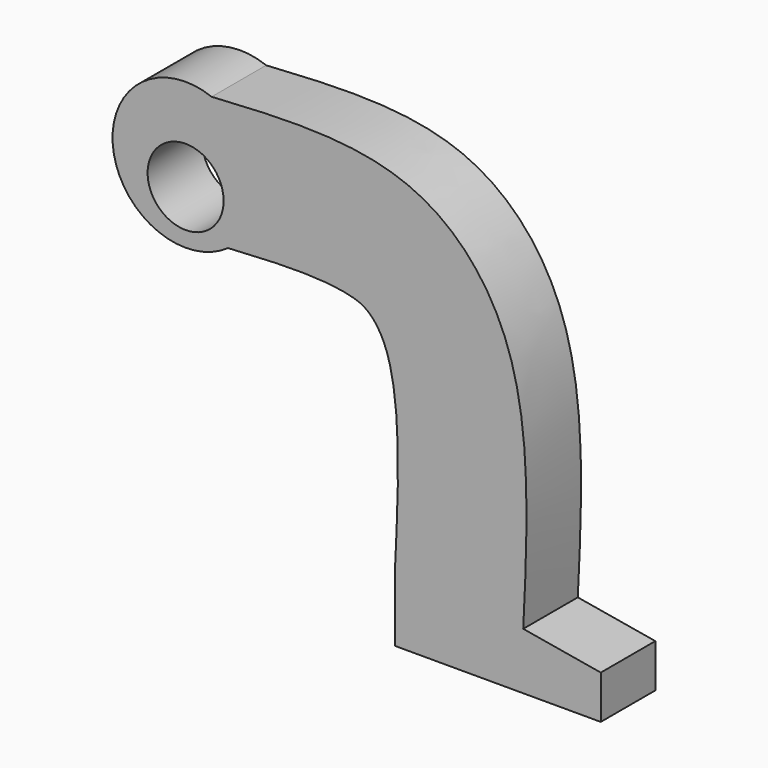
from build123d import *

# Parameters (mm, degrees)
F1_DEPTH = 7
F2_R     = 3.9
F3_DEPTH = 25


# Not quite as in the source:
# - ends of sketch curves that miss each other by under 0.0002 mm in the source are joined
# - the dataset's text gives a spline's control points without its knots; the knots are read off the source's solid


with BuildPart() as f1:
    # F0 (on Front) → F1 (new body)
    with BuildSketch(Plane.XZ):
        with BuildLine():
            add(Edge.make_bspline(
                [(2.6675548526, 7.0095756725), (9.9466486375, 7.453696747), (23.6105158189, 8.2821493946), (35.8507052692, -5.7834758803), (35.0790148845, -21.7545178271), (34.6487350762, -30.6607671082)],
                knots=[0, 0, 0, 0, 0.3351894082, 0.6292627681, 1, 1, 1, 1], degree=3))
            ThreePointArc((2.6675548526, 7.0095756725), (-7.4394221806, -0.9513136277), (4.3455710058, -6.1127745446))
            add(Edge.make_bspline(
                [(4.3455710058, -6.1127745446), (5.3891405614, -6.0498316594), (7.6843362497, -5.9165406912), (10.9253144196, -5.8060227215), (13.8856209942, -5.8700018706), (15.7808027565, -6.0874058733), (16.7453601396, -6.2897087839), (17.1897220211, -6.4084184169), (17.469776248, -6.4959038726), (17.6984548015, -6.5789229449), (17.935730162, -6.6779012945), (18.2137061971, -6.8183248013), (18.5218848655, -7.0140479544), (18.8233111562, -7.2486234624), (19.1262983711, -7.5344088665), (19.4349362667, -7.884892544), (19.7479207593, -8.3124495536), (20.0600135431, -8.8274515425), (20.3124903035, -9.3357541203), (20.505036356, -9.7925679397), (20.6431005208, -10.1598390415), (20.7745963912, -10.5550369644), (20.9490677171, -11.1507905059), (21.1559433245, -12.0126577006), (21.3728446832, -13.2297306672), (21.6070152211, -15.0773377917), (21.7818347688, -17.7706509611), (21.8035125183, -21.4920595704), (21.6778381248, -25.593639044), (21.5366515935, -28.5223388593), (21.4641132996, -30.0237900428)],
                knots=[0.0135442019, 0.0135442019, 0.0135442019, 0.0135442019, 0.0625, 0.125, 0.1875, 0.25, 0.28125, 0.296875, 0.3125, 0.328125, 0.34375, 0.375, 0.40625, 0.4375, 0.46875, 0.5, 0.53125, 0.5625, 0.59375, 0.609375, 0.625, 0.640625, 0.65625, 0.6875, 0.71875, 0.75, 0.8125, 0.875, 0.9375, 1, 1, 1, 1], degree=3))
            Line((21.4641132996, -30.0237900428), (21.4641132996, -36.4838130772))
            Line((21.4641132996, -36.4838130772), (42.605035007, -36.4838130772))
            Line((42.605035007, -36.4838130772), (42.605035007, -32.0257842541))
            Line((42.605035007, -32.0257842541), (34.6487350762, -30.6607671082))
        make_face()
    extrude(amount=F1_DEPTH)

    # F2 (on face) → F3 (cut)
    with BuildSketch(Plane.XZ.offset(7)):
        with Locations((0, -2)):
            Circle(F2_R)
    extrude(amount=-F3_DEPTH, mode=Mode.SUBTRACT)


solid = f1.part
